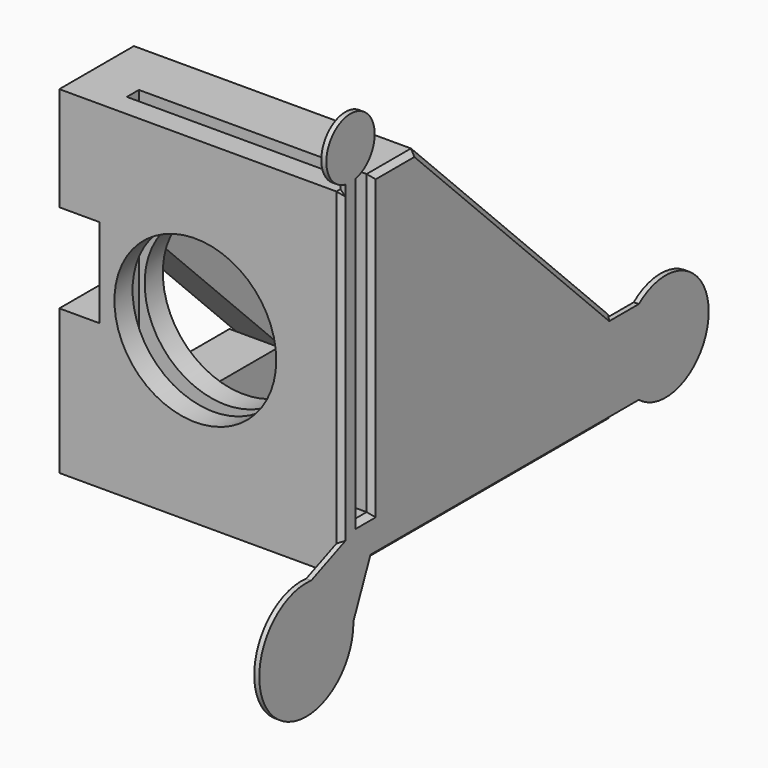
from build123d import *

# Parameters (mm, degrees)
F2_W      = 22.1
F2_H      = 30
F2_R      = 8.03
F2_W_2    = 4.9
F3_DEPTH  = 4
F4_DEPTH  = 6
F6_DEPTH  = 13.5
F7_DEPTH  = 27
F8_DEPTH  = 22.1
F9_DEPTH  = 5.47
F10_R     = 8.03
F11_DEPTH = 6
F13_DEPTH = 22.1
F15_DEPTH = 4
F16_DEPTH = 1
F17_W     = 17.2
F17_H     = 21.2132034356
F18_DEPTH = 4
F19_W     = 1.5
F19_H     = 29.5369624409
F20_DEPTH = 1
F21_SIZE  = 0.5
F23_DEPTH = 0.5


with BuildPart() as f3:
    # F2 (on line) → F3 (new body)
    with BuildSketch(Plane(origin=(0, 0, 0), x_dir=(-1, 0, 0), z_dir=(0, 0.7071067812, 0.7071067812))):
        with Locations((-2.45, 0)):
            Rectangle(F2_W, F2_H)
        Circle(F2_R, mode=Mode.SUBTRACT)
        with Locations((11.05, 0)):
            Rectangle(F2_W_2, F2_H)
    extrude(amount=F3_DEPTH)

    # F2 (on line) → F4 (join)
    with BuildSketch(Plane(origin=(0, 0, 0), x_dir=(-1, 0, 0), z_dir=(0, 0.7071067812, 0.7071067812))):
        with Locations((11.05, 0)):
            Rectangle(F2_W_2, F2_H)
    extrude(amount=-F4_DEPTH)


with BuildPart() as f6:
    # F5 (on face) → F6 (new body)
    with BuildSketch(Plane.YZ.offset(13.5)):
        Polygon((-7.7781745931, 13.8592929113), (13.8592929113, -7.7781745931), (16.687720036, -7.7781745931), (-7.7781745931, 16.687720036), align=None)
    extrude(amount=-F6_DEPTH)

    # F5 (on face) → F7 (join, through all)
    with BuildSketch(Plane.YZ.offset(13.5)):
        Polygon((-11.0308657865, 10.6066017178), (-7.7781745931, 13.8592929113), (-7.7781745931, 16.687720036), (-13.8592929113, 10.6066017178), (-12.3582416429, 9.1055504494), (-11.0308657865, 10.4174916732), align=None)
        Polygon((16.687720036, -16.8492424049), (16.687720036, -7.7781745931), (10.6066017178, -13.8592929113), (9.5965512115, -12.8492424049), (8.6468037432, -12.8492424049), (6.3639610307, -15.1320851174), (4.0811183182, -12.8492424049), (-11.0308657865, -12.8492424049), (-11.0308657865, 2.2627416998), (-15.1320851174, 6.3639610307), (-12.3582416429, 9.1055504494), (-13.8592929113, 10.6066017178), (-7.7781745931, 16.687720036), (-13.8592929113, 16.687720036), (-17.0308657865, 16.687720036), (-17.0308657865, 10.6066017178), (-17.0308657865, -14.8492424049), (-17.0308657865, -16.8492424049), align=None)
        Polygon((16.687720036, -7.7781745931), (13.8592929113, -7.7781745931), (10.6066017178, -11.0308657865), (10.5358910397, -10.9601551084), (9.1216774773, -12.3743686708), (9.5965512115, -12.8492424049), (10.6066017178, -13.8592929113), align=None)
        Polygon((9.5965512115, -12.8492424049), (9.1216774773, -12.3743686708), (8.6468037432, -12.8492424049), align=None)
    extrude(amount=-F7_DEPTH)

    # F5 (on face) → F8 (join, through all)
    with BuildSketch(Plane.YZ.offset(13.5)):
        Polygon((-11.0308657865, 7.7781745931), (-11.0308657865, 10.4174916732), (-12.3582416429, 9.1055504494), align=None)
        Polygon((-11.0308657865, 2.2627416998), (-11.0308657865, 7.7781745931), (-12.3582416429, 9.1055504494), (-15.1320851174, 6.3639610307), align=None)
        Polygon((6.3639610307, -15.1320851174), (8.6468037432, -12.8492424049), (4.0811183182, -12.8492424049), align=None)
    extrude(amount=-F8_DEPTH)

    # F5 (on face) → F9 (join, through all)
    with BuildSketch(Plane.YZ.offset(13.5)):
        Polygon((9.1216774773, -12.3743686708), (10.5358910397, -10.9601551084), (-10.9357578098, 10.5114937411), (-11.0308657865, 10.4174916732), (-11.0308657865, 7.7781745931), align=None)
    extrude(amount=-F9_DEPTH)

    # F10 (on face) → F11 (cut)
    with BuildSketch(Plane.XZ.offset(17.0308657865)):
        Circle(F10_R)
    extrude(amount=-F11_DEPTH, mode=Mode.SUBTRACT)

    # F12 (on face) → F13 (cut, through all)
    with BuildSketch(Plane.YZ.offset(13.5)):
        Polygon((-14.7808657865, 6.711096408), (-13.2808657865, 8.1936545141), (-13.2808657865, 10.0281745931), (-13.8592929113, 10.6066017178), (-13.2808657865, 11.1850288425), (-13.2808657865, 16.687720036), (-13.8592929113, 16.687720036), (-14.7808657865, 16.687720036), align=None)
        Polygon((-13.8592929113, 10.6066017178), (-13.2808657865, 10.0281745931), (-13.2808657865, 11.1850288425), align=None)
        Polygon((-14.7808657865, 6.0127416998), (-13.2808657865, 4.5127416998), (-13.2808657865, 8.1936545141), (-14.7808657865, 6.711096408), align=None)
        Polygon((-14.7808657865, -12.8492424049), (-13.2808657865, -12.8492424049), (-13.2808657865, 4.5127416998), (-14.7808657865, 6.0127416998), align=None)
    extrude(amount=-F13_DEPTH, mode=Mode.SUBTRACT)

    # F14 (on face) → F15 (cut)
    with BuildSketch(Plane(origin=(-13.5, 0, 0), x_dir=(0, -1, 0), z_dir=(-1, 0, 0))):
        Polygon((17.0308657865, 6.3639610307), (15.1320851174, 6.3639610307), (11.0308657865, 2.2627416998), (11.0308657865, -2.4678555783), (17.0308657865, -2.4678555783), align=None)
    extrude(amount=-F15_DEPTH, mode=Mode.SUBTRACT)

    # F5 (on face) → F16 (join)
    with BuildSketch(Plane.YZ.offset(13.5)):
        Polygon((-11.0308657865, 2.2627416998), (-11.0308657865, 7.7781745931), (-12.3582416429, 9.1055504494), (-15.1320851174, 6.3639610307), align=None)
        Polygon((-11.0308657865, 10.6066017178), (-7.7781745931, 13.8592929113), (-7.7781745931, 16.687720036), (-13.8592929113, 10.6066017178), (-12.3582416429, 9.1055504494), (-11.0308657865, 10.4174916732), align=None)
        Polygon((16.687720036, -16.8492424049), (16.687720036, -7.7781745931), (10.6066017178, -13.8592929113), (9.5965512115, -12.8492424049), (8.6468037432, -12.8492424049), (6.3639610307, -15.1320851174), (4.0811183182, -12.8492424049), (-11.0308657865, -12.8492424049), (-11.0308657865, 2.2627416998), (-15.1320851174, 6.3639610307), (-12.3582416429, 9.1055504494), (-13.8592929113, 10.6066017178), (-7.7781745931, 16.687720036), (-13.8592929113, 16.687720036), (-17.0308657865, 16.687720036), (-17.0308657865, 10.6066017178), (-17.0308657865, -14.8492424049), (-17.0308657865, -16.8492424049), align=None)
        Polygon((4.0811183182, -12.8492424049), (-11.0308657865, 2.2627416998), (-11.0308657865, -12.8492424049), align=None)
        Polygon((-11.0308657865, 7.7781745931), (-11.0308657865, 10.4174916732), (-12.3582416429, 9.1055504494), align=None)
        Polygon((8.6468037432, -12.8492424049), (9.1216774773, -12.3743686708), (-11.0308657865, 7.7781745931), (-11.0308657865, 2.2627416998), (4.0811183182, -12.8492424049), align=None)
        Polygon((9.1216774773, -12.3743686708), (10.5358910397, -10.9601551084), (-10.9357578098, 10.5114937411), (-11.0308657865, 10.4174916732), (-11.0308657865, 7.7781745931), align=None)
        Polygon((10.6066017178, -11.0308657865), (13.8592929113, -7.7781745931), (-7.7781745931, 13.8592929113), (-11.0308657865, 10.6066017178), (-10.9357578098, 10.5114937411), (10.5358910397, -10.9601551084), align=None)
        Polygon((-10.6066017178, 10.6066017178), (-7.7781745931, 13.4350288425), (13.4350288425, -7.7781745931), (10.6066017178, -10.6066017178), align=None, mode=Mode.SUBTRACT)
        Polygon((-7.7781745931, 13.8592929113), (13.8592929113, -7.7781745931), (16.687720036, -7.7781745931), (-7.7781745931, 16.687720036), align=None)
        Polygon((6.3639610307, -15.1320851174), (8.6468037432, -12.8492424049), (4.0811183182, -12.8492424049), align=None)
        Polygon((16.687720036, -7.7781745931), (13.8592929113, -7.7781745931), (10.6066017178, -11.0308657865), (10.5358910397, -10.9601551084), (9.1216774773, -12.3743686708), (9.5965512115, -12.8492424049), (10.6066017178, -13.8592929113), align=None)
        Polygon((9.5965512115, -12.8492424049), (9.1216774773, -12.3743686708), (8.6468037432, -12.8492424049), align=None)
        Polygon((13.4350288425, -7.7781745931), (-7.7781745931, 13.4350288425), (-10.6066017178, 10.6066017178), (10.6066017178, -10.6066017178), align=None)
        Polygon((-10.9357578098, 10.5114937411), (-11.0308657865, 10.6066017178), (-11.0308657865, 10.4174916732), align=None)
    extrude(amount=F16_DEPTH)

    # F17 (on face) → F18 (cut, through all)
    with BuildSketch(Plane(origin=(0, 0, -16.8492424049), x_dir=(1, 0, 0), z_dir=(0, 0, -1))):
        Rectangle(F17_W, F17_H)
    extrude(amount=-F18_DEPTH, mode=Mode.SUBTRACT)

    # F19 (on face) → F20 (cut, through all)
    with BuildSketch(Plane.YZ.offset(14.5)):
        with Locations((-14.0308657865, 1.9192388155)):
            Rectangle(F19_W, F19_H)
    extrude(amount=-F20_DEPTH, mode=Mode.SUBTRACT)

    # F21
    f21_edges = [f6.edges().sort_by_distance(p)[0] for p in [
        (14.5, -0.171573, -16.849242),
        (14.5, -17.030866, -0.080761),
        (14.5, -15.905866, 16.68772),
        (14.5, -14.780866, 1.919239),
        (14.5, -14.030866, -12.849242),
        (14.5, -13.280866, 1.919239),
        (14.5, -10.52952, 16.68772),
        (14.5, 4.454773, 4.454773),
        (14.5, 16.68772, -12.313708),
    ]]
    chamfer(f21_edges, length=F21_SIZE)

    # F22 (on face) → F23 (join)
    with BuildSketch(Plane.YZ.offset(14.5)):
        with BuildLine():
            ThreePointArc((-15.2808657865, 17.2535463874), (-13.5740210232, 18.3002614272), (-12.9058657865, 20.187720036))
            ThreePointArc((-12.9058657865, 20.187720036), (-17.7933243953, 22.5195647993), (-16.5308657865, 17.2535463874))
            ThreePointArc((-16.5308657865, 17.2535463874), (-15.9058657865, 17.187720036), (-15.2808657865, 17.2535463874))
        make_face()
        with BuildLine():
            ThreePointArc((-15.2808657865, 17.2535463874), (-15.9058657865, 17.187720036), (-16.5308657865, 17.2535463874))
            Line((-16.5308657865, 17.2535463874), (-16.5308657865, 16.187720036))
            Line((-16.5308657865, 16.187720036), (-15.2808657865, 16.187720036))
            Line((-15.2808657865, 16.187720036), (-15.2808657865, 17.2535463874))
        make_face()
        with BuildLine():
            ThreePointArc((-15.5444476146, -21.3166986959), (-17.0770379924, -17.4773914659), (-20.7671737825, -15.6140581293))
            ThreePointArc((-20.7671737825, -15.6140581293), (-25.727715353, -25.3283540085), (-15.5434902172, -21.422451362))
            ThreePointArc((-15.5434902172, -21.422451362), (-15.5437295714, -21.3695728621), (-15.5444476146, -21.3166986959))
        make_face()
        with BuildLine():
            Line((-16.5308657865, -16.3492424049), (-16.5308657865, -13.8718290254))
            Line((-16.5308657865, -13.8718290254), (-20.7671737825, -15.6140581293))
            ThreePointArc((-20.7671737825, -15.6140581293), (-17.0770379924, -17.4773914659), (-15.5444476146, -21.3166986959))
            Line((-15.5444476146, -21.3166986959), (-13.4268440306, -16.3492424049))
            Line((-13.4268440306, -16.3492424049), (-16.5308657865, -16.3492424049))
        make_face()
        with BuildLine():
            ThreePointArc((19.8610443441, -7.9852813742), (17.8439636615, -12.1672618896), (19.8610443441, -16.3492424049))
            ThreePointArc((19.8610443441, -16.3492424049), (25.5092268479, -16.9804041389), (28.5314764105, -12.1672618896))
            ThreePointArc((28.5314764105, -12.1672618896), (25.5092268479, -7.3541196403), (19.8610443441, -7.9852813742))
        make_face()
        with BuildLine():
            Line((16.187720036, -7.9852813742), (16.187720036, -16.3492424049))
            Line((16.187720036, -16.3492424049), (19.8610443441, -16.3492424049))
            ThreePointArc((19.8610443441, -16.3492424049), (17.8439636615, -12.1672618896), (19.8610443441, -7.9852813742))
            Line((19.8610443441, -7.9852813742), (16.187720036, -7.9852813742))
        make_face()
    extrude(amount=-F23_DEPTH)


solid = Compound([f3.part, f6.part])
